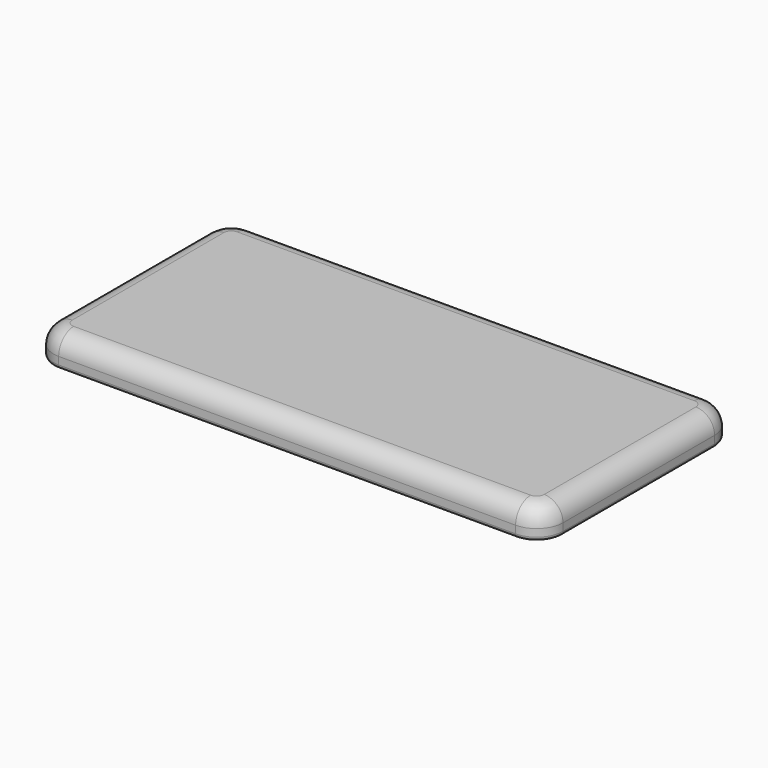
from build123d import *

# Parameters (mm, degrees)
F0_W         = 135.5529725552
F0_H         = 64.4017234445
F1_DEPTH     = 8
F2_R         = 5
F3_T1_DEPTH  = 25.5
F3_T4_ANGLE  = 90
F3_T6_ANGLE  = 90
F3_T8_ANGLE  = 90
F3_T10_ANGLE = 90
F4_R         = 1
F5_W         = 105.8298870921
F5_H         = 54.4540472329
F6_DEPTH     = 1


# Not quite as in the source:
# - a fillet or chamfer that OpenCascade refuses, or shapes differently, is made with other operations: its cross-section is extruded or revolved along the edge and cut away or added


with BuildPart() as f1:
    # F0 (on Top) → F1 (new body)
    with BuildSketch(Plane.XY):
        Rectangle(F0_W, F0_H)
    extrude(amount=F1_DEPTH)

    # F2
    f2_edges = [f1.edges().sort_by_distance(p)[0] for p in [
        (0, 32.200862, 8),
        (-67.776486, 0, 8),
        (0, -32.200862, 8),
        (67.776486, 0, 8),
    ]]
    fillet(f2_edges, radius=F2_R)

    # F3: fillet of radius 7 on 4 edges, made by hand

    # F3_s2 → F3_t1 (cut)
    with BuildSketch(Plane.XY.offset(-17.5)):
        with BuildLine():
            ThreePointArc((-67.7764862776, -25.2008617222), (-65.7262337459, -30.1506091905), (-60.7764862776, -32.2008617222))
            Line((-60.7764862776, -32.2008617222), (-67.7764862776, -32.2008617222))
            Line((-67.7764862776, -32.2008617222), (-67.7764862776, -25.2008617222))
        make_face()
        with BuildLine():
            ThreePointArc((60.7764862776, -32.2008617222), (65.7262337459, -30.1506091905), (67.7764862776, -25.2008617222))
            Line((67.7764862776, -25.2008617222), (67.7764862776, -32.2008617222))
            Line((67.7764862776, -32.2008617222), (60.7764862776, -32.2008617222))
        make_face()
        with BuildLine():
            ThreePointArc((60.7764862776, 32.2008617222), (65.7262337459, 30.1506091905), (67.7764862776, 25.2008617222))
            Line((67.7764862776, 25.2008617222), (67.7764862776, 32.2008617222))
            Line((67.7764862776, 32.2008617222), (60.7764862776, 32.2008617222))
        make_face()
        with BuildLine():
            ThreePointArc((-67.7764862776, 25.2008617222), (-65.7262337459, 30.1506091905), (-60.7764862776, 32.2008617222))
            Line((-60.7764862776, 32.2008617222), (-67.7764862776, 32.2008617222))
            Line((-67.7764862776, 32.2008617222), (-67.7764862776, 25.2008617222))
        make_face()
    extrude(amount=F3_T1_DEPTH, mode=Mode.SUBTRACT)

    # F3_s3 → F3_t4 (revolve, cut)
    with BuildSketch(Plane.YZ.offset(-60.7764862776)):
        with BuildLine():
            ThreePointArc((27.2008617222, 8), (30.7363956282, 6.5355339059), (32.2008617222, 3))
            Line((32.2008617222, 3), (32.2008617222, 8))
            Line((32.2008617222, 8), (27.2008617222, 8))
        make_face()
    revolve(axis=Axis((-60.7764862776, 25.2008617222, 8), (0, 0, 1)), revolution_arc=F3_T4_ANGLE, mode=Mode.SUBTRACT)

    # F3_s5 → F3_t6 (revolve, cut)
    with BuildSketch(Plane.XZ.offset(-25.2008617222)):
        with BuildLine():
            ThreePointArc((62.7764862776, 8), (66.3120201835, 6.5355339059), (67.7764862776, 3))
            Line((67.7764862776, 3), (67.7764862776, 8))
            Line((67.7764862776, 8), (62.7764862776, 8))
        make_face()
    revolve(axis=Axis((60.7764862776, 25.2008617222, 8), (0, 0, 1)), revolution_arc=F3_T6_ANGLE, mode=Mode.SUBTRACT)

    # F3_s7 → F3_t8 (revolve, cut)
    with BuildSketch(Plane.YZ.offset(60.7764862776)):
        with BuildLine():
            ThreePointArc((-27.2008617222, 8), (-30.7363956282, 6.5355339059), (-32.2008617222, 3))
            Line((-32.2008617222, 3), (-32.2008617222, 8))
            Line((-32.2008617222, 8), (-27.2008617222, 8))
        make_face()
    revolve(axis=Axis((60.7764862776, -25.2008617222, 8), (0, 0, 1)), revolution_arc=F3_T8_ANGLE, mode=Mode.SUBTRACT)

    # F3_s9 → F3_t10 (revolve, cut)
    with BuildSketch(Plane.XZ.offset(25.2008617222)):
        with BuildLine():
            ThreePointArc((-62.7764862776, 8), (-66.3120201835, 6.5355339059), (-67.7764862776, 3))
            Line((-67.7764862776, 3), (-67.7764862776, 8))
            Line((-67.7764862776, 8), (-62.7764862776, 8))
        make_face()
    revolve(axis=Axis((-60.7764862776, -25.2008617222, 8), (0, 0, 1)), revolution_arc=F3_T10_ANGLE, mode=Mode.SUBTRACT)

    # F4
    f4_edges = [f1.edges().sort_by_distance(p)[0] for p in [
        (0, -32.200862, 0),
        (-67.776486, 0, 0),
    ]]
    fillet(f4_edges, radius=F4_R)

    # F5 (on face) → F6 (cut)
    with BuildSketch(Plane(origin=(0, 0, 0), x_dir=(1, 0, 0), z_dir=(0, 0, -1))):
        Rectangle(F5_W, F5_H)
    extrude(amount=-F6_DEPTH, mode=Mode.SUBTRACT)


solid = f1.part
